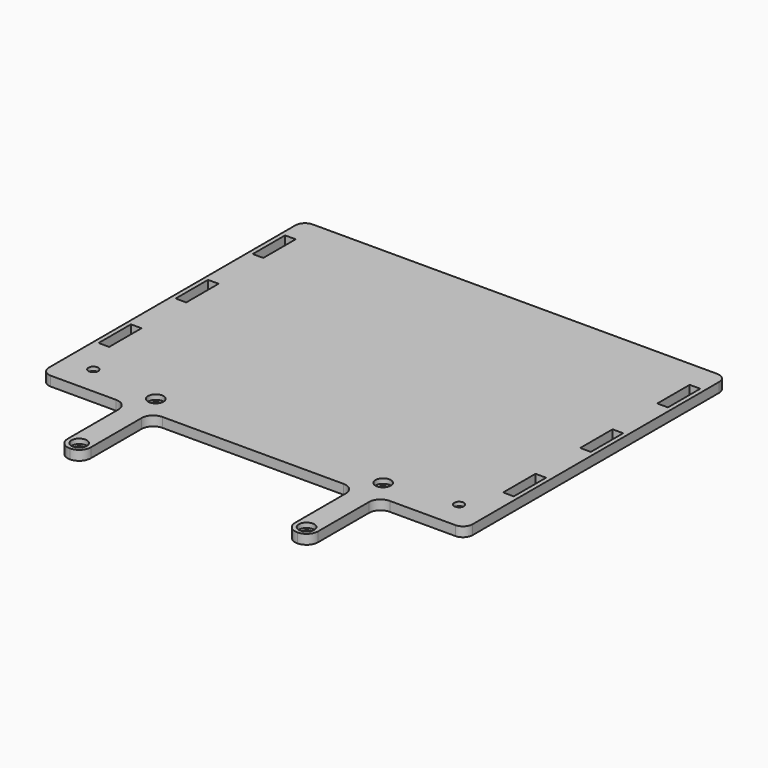
from build123d import *

# Parameters (mm, degrees)
F0_W      = 220
F0_H      = 170
F0_W_2    = 200
F0_H_2    = 150
F1_DEPTH  = 5
F2_W      = 5.5
F2_H      = 21
F3_DEPTH  = 25
F4_W      = 12
F4_H      = 5
F5_DEPTH  = 45
F6_R      = 2.2
F7_DEPTH  = 25
F8_R      = 5.99999
F9_R      = 6
F10_R     = 4
F11_DEPTH = 2.5
F13_R     = 5
F15_DEPTH = 3
F12_R     = 2.5
F16_DEPTH = 3


# Not quite as in the source:
# - a fillet or chamfer is up to 0.001 mm smaller than in the source, because OpenCascade refuses the exact size


with BuildPart() as f1:
    # F0 (on Top) → F1 (new body)
    with BuildSketch(Plane.XY):
        Rectangle(F0_W, F0_H)
        Rectangle(F0_W_2, F0_H_2, mode=Mode.SUBTRACT)
        Rectangle(F0_W_2, F0_H_2)
    extrude(amount=F1_DEPTH)

    # F2 (on face) → F3 (cut)
    with BuildSketch(Plane.XY.offset(5)):
        with Locations((-105, 60)):
            Rectangle(F2_W, F2_H)
        with Locations((-105, 10)):
            Rectangle(F2_W, F2_H)
        with Locations((-105, -40)):
            Rectangle(F2_W, F2_H)
        with Locations((105, 60)):
            Rectangle(F2_W, F2_H)
        with Locations((105, 10)):
            Rectangle(F2_W, F2_H)
        with Locations((105, -40)):
            Rectangle(F2_W, F2_H)
    extrude(amount=-F3_DEPTH, mode=Mode.SUBTRACT)

    # F4 (on face) → F5 (join)
    with BuildSketch(Plane.XZ.offset(85)):
        with Locations((59, 2.5)):
            Rectangle(F4_W, F4_H)
        with Locations((-59, 2.5)):
            Rectangle(F4_W, F4_H)
    extrude(amount=F5_DEPTH)

    # F6 (on face) → F7 (cut)
    with BuildSketch(Plane.XY.offset(5)):
        with Locations((-59, -74.3)):
            Circle(F6_R)
        with Locations((-59, -124)):
            Circle(F6_R)
        with Locations((59, -74.3)):
            Circle(F6_R)
        with Locations((59, -124)):
            Circle(F6_R)
    extrude(amount=-F7_DEPTH, mode=Mode.SUBTRACT)

    # F8 (radius 6 in the source; OpenCascade refuses exactly that, so slightly less here)
    f8_edges = [f1.edges().sort_by_distance(p)[0] for p in [
        (-65, -130, 2.5),
        (-53, -130, 2.5),
        (53, -130, 2.5),
        (65, -130, 2.5),
    ]]
    fillet(f8_edges, radius=F8_R)

    # F9
    f9_edges = [f1.edges().sort_by_distance(p)[0] for p in [
        (-65, -85, 2.5),
        (-53, -85, 2.5),
        (53, -85, 2.5),
        (65, -85, 2.5),
    ]]
    fillet(f9_edges, radius=F9_R)

    # F10 (on face) → F11 (cut)
    with BuildSketch(Plane.XY.offset(5)):
        with Locations((-59, -124)):
            Circle(F10_R)
        with Locations((-59, -74.3)):
            Circle(F10_R)
        with Locations((59, -74.3)):
            Circle(F10_R)
        with Locations((59, -124)):
            Circle(F10_R)
    extrude(amount=-F11_DEPTH, mode=Mode.SUBTRACT)

    # F13
    f13_edges = [f1.edges().sort_by_distance(p)[0] for p in [
        (-110, -85, 2.5),
        (110, -85, 2.5),
        (110, 85, 2.5),
        (-110, 85, 2.5),
    ]]
    fillet(f13_edges, radius=F13_R)

    # F14 (on face) → F15 (cut)
    with BuildSketch(Plane.XY):
        Polygon((-98.42, -67.8992740578), (-98.42, -71.9407259422), (-94.92, -73.9614518843), (-91.42, -71.9407259422), (-91.42, -67.8992740578), (-94.92, -65.8785481157), align=None)
        Polygon((98.42, -71.9407259422), (98.42, -67.8992740578), (94.92, -65.8785481157), (91.42, -67.8992740578), (91.42, -71.9407259422), (94.92, -73.9614518843), align=None)
    extrude(amount=F15_DEPTH, mode=Mode.SUBTRACT)

    # F12 (on face) → F16 (cut)
    with BuildSketch(Plane.XY.offset(5)):
        with Locations((94.92, -69.92)):
            Circle(F12_R)
        with Locations((-94.92, -69.92)):
            Circle(F12_R)
    extrude(amount=-F16_DEPTH, mode=Mode.SUBTRACT)


solid = f1.part
